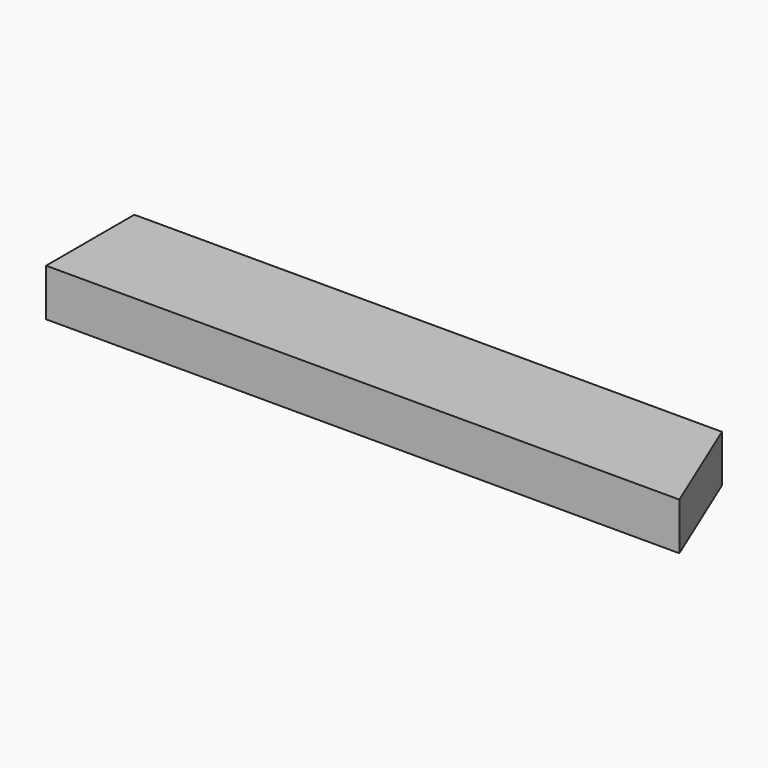
from build123d import *

# Parameters (mm, degrees)
F0_W     = 510.4854979371
F0_H     = 88.9
F1_DEPTH = 38.1
F2_SIZE2 = 36.823576
F2_SIZE  = 88.89999


# Not quite as in the source:
# - a fillet or chamfer is up to 0.001 mm smaller than in the source, because OpenCascade refuses the exact size


with BuildPart() as f1:
    # F0 (on Top) → F1 (new body)
    with BuildSketch(Plane.XY):
        with Locations((255.2427489686, 44.45)):
            Rectangle(F0_W, F0_H)
    extrude(amount=F1_DEPTH)

    # F2 (size 88.9 and 36.823585695 in the source; OpenCascade refuses exactly that, so slightly less here)
    f2_edges = [f1.edges().sort_by_distance(p)[0] for p in [
        (510.485498, 88.9, 19.05),
    ]]
    f2_side = f1.faces().sort_by_distance((510.485498, 44.45, 19.05))[0]
    chamfer(f2_edges, length=F2_SIZE, length2=F2_SIZE2, reference=f2_side)


solid = f1.part
